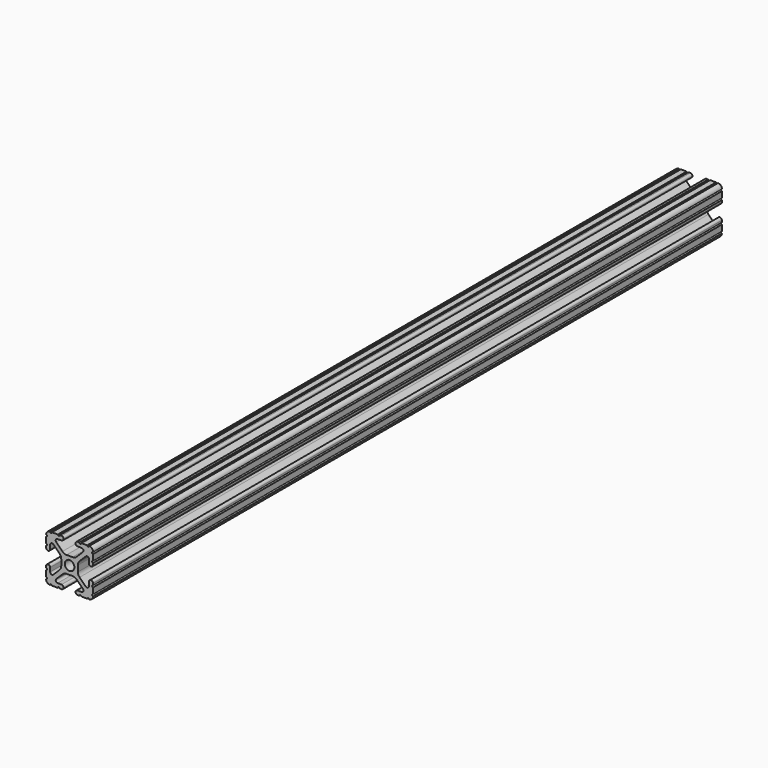
from build123d import *

# Parameters (mm, degrees)
F1_DEPTH = 425


# Not quite as in the source:
# - ends of sketch curves that miss each other by under 0.0002 mm in the source are joined


with BuildPart() as f1:
    # F0 (on Front) → F1 (new body)
    with BuildSketch(Plane.XZ):
        with BuildLine():
            ThreePointArc((-12.7, -9.5504), (-12.1920000057, -10.0583238), (-12.6998476, -10.5663999771))
            ThreePointArc((-12.6998476, -10.5663999771), (-12.0825225161, -12.0825225161), (-10.5664000074, -12.6998469825))
            ThreePointArc((-10.5664000074, -12.6998469825), (-10.0583238, -12.1920000057), (-9.5504, -12.7))
            Line((-9.5504, -12.7), (-6.3330836, -12.7))
            ThreePointArc((-6.3330836, -12.7), (-5.8250836, -12.192), (-5.3170836, -12.7))
            Line((-5.3170836, -12.7), (-4.3434, -12.7))
            ThreePointArc((-4.3434, -12.7), (-3.2385, -11.5951), (-4.3434, -10.4902))
            Line((-4.3434, -10.4902), (-6.4747902, -10.4902))
            ThreePointArc((-6.4747902, -10.4902), (-7.413451805, -9.8630063673), (-7.1932106897, -8.7557795103))
            Line((-7.1932106897, -8.7557795103), (-3.8631622, -5.4257448))
            ThreePointArc((-3.8631622, -5.4257448), (-2.8331268978, -4.7374824843), (-1.618107, -4.4958))
            Line((-1.618107, -4.4958), (1.618107, -4.4958))
            ThreePointArc((1.618107, -4.4958), (2.8331268978, -4.7374824843), (3.8631710303, -5.4257359697))
            Line((3.8631710303, -5.4257359697), (7.1932038, -8.7557864))
            ThreePointArc((7.1932038, -8.7557864), (7.413451805, -9.8630063673), (6.4747902, -10.4902))
            Line((6.4747902, -10.4902), (4.3434, -10.4902))
            ThreePointArc((4.3434, -10.4902), (3.2385, -11.5951), (4.3434, -12.7))
            Line((4.3434, -12.7), (5.3170836, -12.7))
            ThreePointArc((5.3170836, -12.7), (5.8250836, -12.192), (6.3330836, -12.7))
            Line((6.3330836, -12.7), (9.5504, -12.7))
            ThreePointArc((9.5504, -12.7), (10.0583238, -12.1920000057), (10.5663999771, -12.6998476))
            ThreePointArc((10.5663999771, -12.6998476), (12.0825225161, -12.0825225161), (12.6998469825, -10.5664000074))
            ThreePointArc((12.6998469825, -10.5664000074), (12.1920000057, -10.0583238), (12.7, -9.5504))
            Line((12.7, -9.5504), (12.7, -6.3330836))
            ThreePointArc((12.7, -6.3330836), (12.192, -5.8250836), (12.7, -5.3170836))
            Line((12.7, -5.3170836), (12.7, -4.3434))
            ThreePointArc((12.7, -4.3434), (11.5951, -3.2385), (10.4902, -4.3434))
            Line((10.4902, -4.3434), (10.4902, -6.4747902))
            ThreePointArc((10.4902, -6.4747902), (9.8630063673, -7.413451805), (8.7557795103, -7.1932106897))
            Line((8.7557795103, -7.1932106897), (5.4257448, -3.8631622))
            ThreePointArc((5.4257448, -3.8631622), (4.7374824843, -2.8331268978), (4.4958, -1.618107))
            Line((4.4958, -1.618107), (4.4958, 1.618107))
            ThreePointArc((4.4958, 1.618107), (4.7374824843, 2.8331268978), (5.4257359697, 3.8631710303))
            Line((5.4257359697, 3.8631710303), (8.7557864, 7.1932038))
            ThreePointArc((8.7557864, 7.1932038), (9.8630063673, 7.413451805), (10.4902, 6.4747902))
            Line((10.4902, 6.4747902), (10.4902, 4.3434))
            ThreePointArc((10.4902, 4.3434), (11.5951, 3.2385), (12.7, 4.3434))
            Line((12.7, 4.3434), (12.7, 5.3170836))
            ThreePointArc((12.7, 5.3170836), (12.192, 5.8250836), (12.7, 6.3330836))
            Line((12.7, 6.3330836), (12.7, 9.5504))
            ThreePointArc((12.7, 9.5504), (12.1920000057, 10.0583238), (12.6998476, 10.5663999771))
            ThreePointArc((12.6998476, 10.5663999771), (12.0825225161, 12.0825225161), (10.5664000074, 12.6998469825))
            ThreePointArc((10.5664000074, 12.6998469825), (10.0583238, 12.1920000057), (9.5504, 12.7))
            Line((9.5504, 12.7), (6.3330836, 12.7))
            ThreePointArc((6.3330836, 12.7), (5.8250836, 12.192), (5.3170836, 12.7))
            Line((5.3170836, 12.7), (4.3434, 12.7))
            ThreePointArc((4.3434, 12.7), (3.2385, 11.5951), (4.3434, 10.4902))
            Line((4.3434, 10.4902), (6.4747902, 10.4902))
            ThreePointArc((6.4747902, 10.4902), (7.413451805, 9.8630063673), (7.1932106897, 8.7557795103))
            Line((7.1932106897, 8.7557795103), (3.8631622, 5.4257448))
            ThreePointArc((3.8631622, 5.4257448), (2.8331268978, 4.7374824843), (1.618107, 4.4958))
            Line((1.618107, 4.4958), (-1.618107, 4.4958))
            ThreePointArc((-1.618107, 4.4958), (-2.8331268978, 4.7374824843), (-3.8631710303, 5.4257359697))
            Line((-3.8631710303, 5.4257359697), (-7.1932038, 8.7557864))
            ThreePointArc((-7.1932038, 8.7557864), (-7.413451805, 9.8630063673), (-6.4747902, 10.4902))
            Line((-6.4747902, 10.4902), (-4.3434, 10.4902))
            ThreePointArc((-4.3434, 10.4902), (-3.2385, 11.5951), (-4.3434, 12.7))
            Line((-4.3434, 12.7), (-5.3170836, 12.7))
            ThreePointArc((-5.3170836, 12.7), (-5.8250836, 12.192), (-6.3330836, 12.7))
            Line((-6.3330836, 12.7), (-9.5504, 12.7))
            ThreePointArc((-9.5504, 12.7), (-10.0583238, 12.1920000057), (-10.5663999771, 12.6998476))
            ThreePointArc((-10.5663999771, 12.6998476), (-12.0825225161, 12.0825225161), (-12.6998469825, 10.5664000074))
            ThreePointArc((-12.6998469825, 10.5664000074), (-12.1920000057, 10.0583238), (-12.7, 9.5504))
            Line((-12.7, 9.5504), (-12.7, 6.3330836))
            ThreePointArc((-12.7, 6.3330836), (-12.192, 5.8250836), (-12.7, 5.3170836))
            Line((-12.7, 5.3170836), (-12.7, 4.3434))
            ThreePointArc((-12.7, 4.3434), (-11.5951, 3.2385), (-10.4902, 4.3434))
            Line((-10.4902, 4.3434), (-10.4902, 6.4747902))
            ThreePointArc((-10.4902, 6.4747902), (-9.8630063673, 7.413451805), (-8.7557795103, 7.1932106897))
            Line((-8.7557795103, 7.1932106897), (-5.4257448, 3.8631622))
            ThreePointArc((-5.4257448, 3.8631622), (-4.7374824843, 2.8331268978), (-4.4958, 1.618107))
            Line((-4.4958, 1.618107), (-4.4958, -1.618107))
            ThreePointArc((-4.4958, -1.618107), (-4.7374824843, -2.8331268978), (-5.4257359697, -3.8631710303))
            Line((-5.4257359697, -3.8631710303), (-8.7557864, -7.1932038))
            ThreePointArc((-8.7557864, -7.1932038), (-9.8630063673, -7.413451805), (-10.4902, -6.4747902))
            Line((-10.4902, -6.4747902), (-10.4902, -4.3434))
            ThreePointArc((-10.4902, -4.3434), (-11.5951, -3.2385), (-12.7, -4.3434))
            Line((-12.7, -4.3434), (-12.7, -5.3170836))
            ThreePointArc((-12.7, -5.3170836), (-12.192, -5.8250836), (-12.7, -6.3330836))
            Line((-12.7, -6.3330836), (-12.7, -9.5504))
        make_face()
        with BuildLine():
            ThreePointArc((-2.6035, 0), (0, 2.6035), (2.6035, 0))
            ThreePointArc((2.6035, 0), (0, -2.6035), (-2.6035, 0))
        make_face(mode=Mode.SUBTRACT)
    extrude(amount=F1_DEPTH)


solid = f1.part
